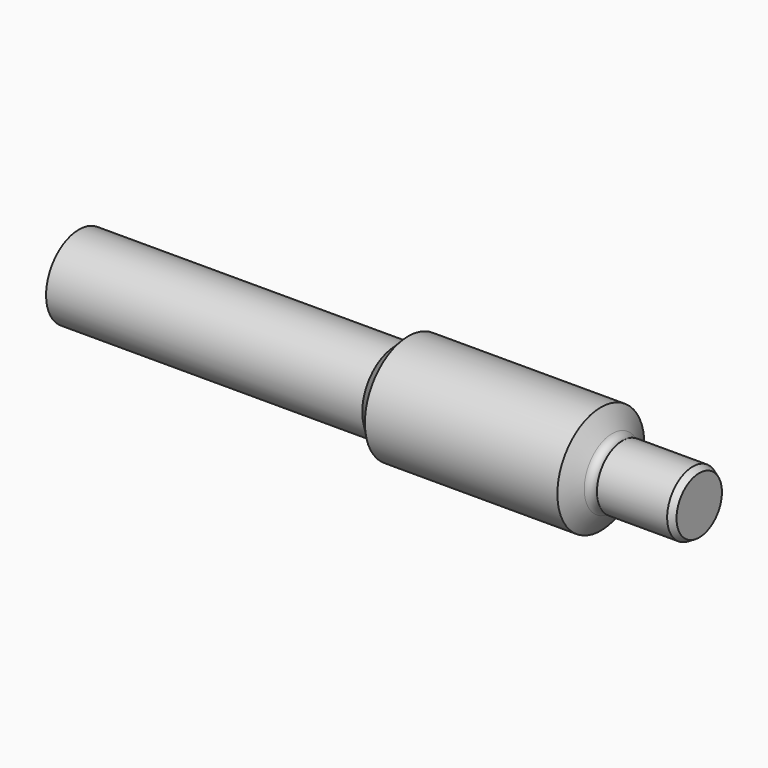
from build123d import *


# Not quite as in the source:
# - a feature names something its author has since deleted; it is built from what else it names


with BuildPart() as f1:
    # F0 (on Front) → F1 (revolve)
    with BuildSketch(Plane.XZ):
        with BuildLine():
            Line((73.9128874429, 9.6128874429), (0, 9.6128874429))
            Line((0, 9.6128874429), (0, 0))
            Line((0, 0), (145, 0))
            Line((145, 0), (145, 6.6339745962))
            Line((145, 6.6339745962), (143.5, 7.5))
            Line((143.5, 7.5), (127.0839127162, 7.5))
            ThreePointArc((127.0839127162, 7.5), (125.7245645959, 7.307737003), (124.6327172275, 8.14))
            Line((124.6327172275, 8.14), (122, 12.7))
            Line((122, 12.7), (77, 12.7))
            Line((77, 12.7), (73.9128874429, 9.6128874429))
        make_face()
    revolve(axis=Axis((72.5, 0, 0), (1, 0, 0)))


solid = f1.part
